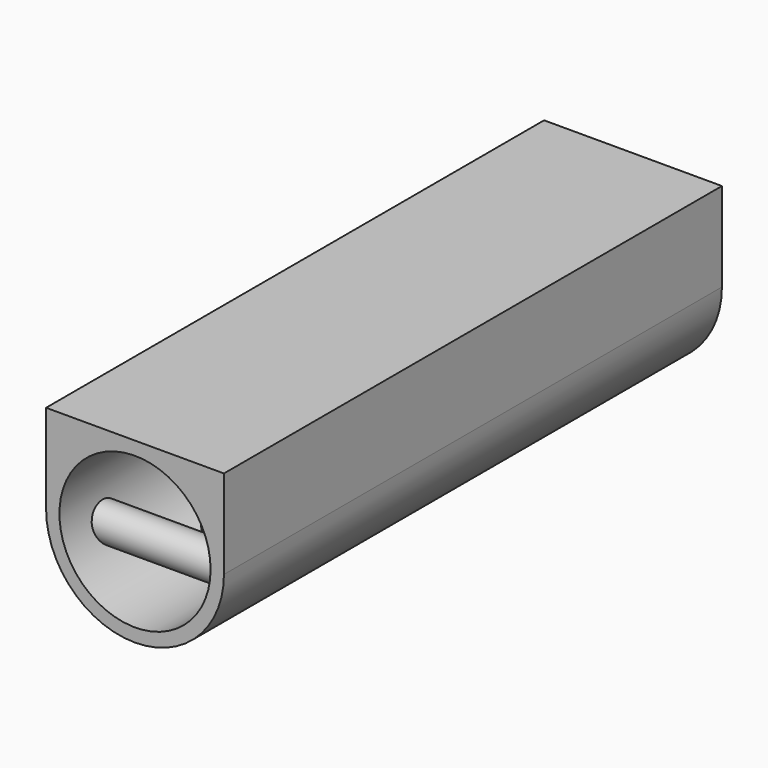
from build123d import *

# Parameters (mm, degrees)
F1_R     = 1
F2_DEPTH = 4.25
F0_R     = 4.25
F0_R_2   = 0.5
F3_DEPTH = 20
F4_DEPTH = 35
F5_DEPTH = 25
F6_R     = 4


with BuildPart() as f2:
    # F1 (on Right) → F2 (new body, symmetric)
    with BuildSketch(Plane.YZ):
        with Locations((-32, 3.5)):
            Circle(F1_R)
    extrude(amount=F2_DEPTH, both=True)


with BuildPart() as f2b:
    # F1 (on Right) → F2, piece 2 (new body, symmetric)
    with BuildSketch(Plane.YZ):
        Polygon((-28.2223820686, 0.75), (-20, 0.75), (-20, 7.25), align=None)
    extrude(amount=F2_DEPTH, both=True)

    # F0 (on Front) → F5 (cut)
    with BuildSketch(Plane.XZ):
        with Locations((0, 5)):
            Circle(F0_R_2)
    extrude(amount=F5_DEPTH, mode=Mode.SUBTRACT)

    # F6
    f6_edges = [f2b.edges().sort_by_distance(p)[0] for p in [
        (-4.25, -24.111191, 0.75),
        (4.25, -24.111191, 0.75),
    ]]
    fillet(f6_edges, radius=F6_R)


with BuildPart() as f3:
    # F0 (on Front) → F3 (new body)
    with BuildSketch(Plane.XZ):
        with Locations((0, 5)):
            Circle(F0_R)
        with Locations((0, 5)):
            Circle(F0_R_2, mode=Mode.SUBTRACT)
    extrude(amount=F3_DEPTH)

    # F0 (on Front) → F4 (join)
    with BuildSketch(Plane.XZ):
        with BuildLine():
            ThreePointArc((-5, 5), (0, 0), (5, 5))
            ThreePointArc((5, 5), (3.5355339059, 8.5355339059), (0, 10))
            ThreePointArc((0, 10), (-3.5355339059, 8.5355339059), (-5, 5))
        make_face()
        with Locations((0, 5)):
            Circle(F0_R, mode=Mode.SUBTRACT)
        with BuildLine():
            ThreePointArc((0, 10), (3.5355339059, 8.5355339059), (5, 5))
            Line((5, 5), (5, 10))
            Line((5, 10), (0, 10))
        make_face()
        with BuildLine():
            ThreePointArc((-5, 5), (-3.5355339059, 8.5355339059), (0, 10))
            Line((0, 10), (-5, 10))
            Line((-5, 10), (-5, 5))
        make_face()
    extrude(amount=F4_DEPTH)


solid = Compound([f2.part, f2b.part, f3.part])
